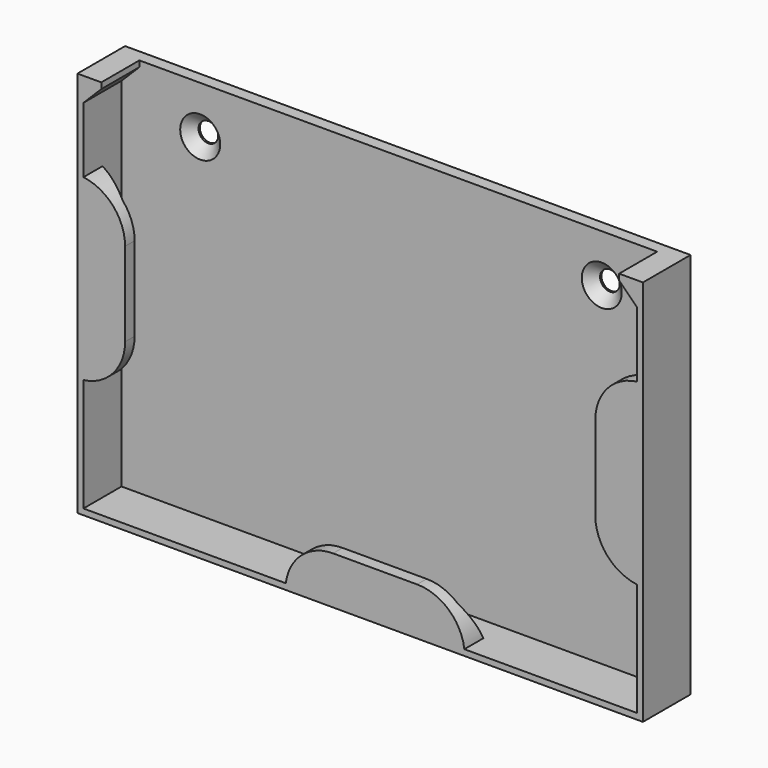
from build123d import *

# Parameters (mm, degrees)
F0_W            = 95
F0_H            = 65
F1_DEPTH        = 10
F2_W            = 93
F2_H            = 63
F3_DEPTH        = 8
F4_W            = 8
F4_H            = 30
F4_W_2          = 30
F4_H_2          = 8
F5_DEPTH        = 2
F6_T1_DEPTH     = 21.843134833
F6_T6_DEPTH     = 41.686269666
F6_T11_DEPTH    = 41.686269666
F7_C1_SIZE2     = 2
F7_C1_SIZE      = 5
F7_C2_SIZE2     = 5
F7_C2_SIZE      = 2
F7_C3_SIZE2     = 2
F7_C3_SIZE      = 5
F8_W            = 87
F8_H            = 8
F9_DEPTH        = 10
F10_SIZE        = 2.99999
F12_D           = 3.3
F12_CSINK_D     = 6.72
F12_CSINK_ANGLE = 90


# Not quite as in the source:
# - a fillet or chamfer that OpenCascade refuses, or shapes differently, is made with other operations: its cross-section is extruded or revolved along the edge and cut away or added
# - a fillet or chamfer is up to 0.001 mm smaller than in the source, because OpenCascade refuses the exact size


with BuildPart() as f1:
    # F0 (on Front) → F1 (new body)
    with BuildSketch(Plane.XZ):
        Rectangle(F0_W, F0_H)
    extrude(amount=F1_DEPTH)

    # F2 (on face) → F3 (cut)
    with BuildSketch(Plane.XZ.offset(10)):
        Rectangle(F2_W, F2_H)
    extrude(amount=-F3_DEPTH, mode=Mode.SUBTRACT)

    # F4 (on face) → F5 (join)
    with BuildSketch(Plane.XZ.offset(10)):
        with Locations((-43.5, 2.5)):
            Rectangle(F4_W, F4_H)
        with Locations((43.5, 2.5)):
            Rectangle(F4_W, F4_H)
        with Locations((2.5, -28.5)):
            Rectangle(F4_W_2, F4_H_2)
    extrude(amount=-F5_DEPTH)

    # F6: fillet of radius 8 on 6 edges, made by hand

    # F6_s2 → F6_t1 (cut)
    with BuildSketch(Plane.XZ.offset(8)):
        with BuildLine():
            ThreePointArc((-39.5, -4.5627460668), (-41.5, -9.8542486889), (-46.5, -12.5))
            Line((-46.5, -12.5), (-39.5, -12.5))
            Line((-39.5, -12.5), (-39.5, -4.5627460668))
        make_face()
        with BuildLine():
            ThreePointArc((-46.5, 17.5), (-41.5, 14.8542486889), (-39.5, 9.5627460668))
            Line((-39.5, 9.5627460668), (-39.5, 17.5))
            Line((-39.5, 17.5), (-46.5, 17.5))
        make_face()
        with BuildLine():
            ThreePointArc((-12.5, -31.5), (-9.8542486889, -26.5), (-4.5627460668, -24.5))
            Line((-4.5627460668, -24.5), (-12.5, -24.5))
            Line((-12.5, -24.5), (-12.5, -31.5))
        make_face()
        with BuildLine():
            ThreePointArc((9.5627460668, -24.5), (14.8542486889, -26.5), (17.5, -31.5))
            Line((17.5, -31.5), (17.5, -24.5))
            Line((17.5, -24.5), (9.5627460668, -24.5))
        make_face()
    extrude(amount=F6_T1_DEPTH, mode=Mode.SUBTRACT)


with BuildPart() as f6_tool4:
    # F6_s5 → F6_t6 (new body)
    with BuildSketch(Plane.XZ.offset(29.843134833)):
        with BuildLine():
            ThreePointArc((39.5, 9.5627460668), (41.5, 14.8542486889), (46.5, 17.5))
            Line((46.5, 17.5), (39.5, 17.5))
            Line((39.5, 17.5), (39.5, 9.5627460668))
        make_face()
    extrude(amount=-F6_T6_DEPTH)

    split(bisect_by=Plane.XZ.offset(2), keep=Keep.TOP)


with BuildPart() as f1_1:
    add(f1.part)

    # F6_t3: cut F6_tool4
    add(f6_tool4.part, mode=Mode.SUBTRACT)


with BuildPart() as f6_tool9:
    # F6_s10 → F6_t11 (new body)
    with BuildSketch(Plane.XZ.offset(29.843134833)):
        with BuildLine():
            ThreePointArc((46.5, -12.5), (41.5, -9.8542486889), (39.5, -4.5627460668))
            Line((39.5, -4.5627460668), (39.5, -12.5))
            Line((39.5, -12.5), (46.5, -12.5))
        make_face()
    extrude(amount=-F6_T11_DEPTH)

    split(bisect_by=Plane.XZ.offset(2), keep=Keep.TOP)


with BuildPart() as f1_2:
    add(f1_1.part)

    # F6_t8: cut F6_tool9
    add(f6_tool9.part, mode=Mode.SUBTRACT)

    # F7: chamfer of 2 x 5 on 3 edges, made by hand

    # F7_c1
    f7_c1_edges = [f1_2.edges().sort_by_distance(p)[0] for p in [
        (2.5, -8, -31.5),
    ]]
    f7_c1_side = f1_2.faces().sort_by_distance((2.5, -8, -31.46))[0]
    chamfer(f7_c1_edges, length=F7_C1_SIZE, length2=F7_C1_SIZE2, reference=f7_c1_side)

    # F7_c2
    f7_c2_edges = [f1_2.edges().sort_by_distance(p)[0] for p in [
        (-46.5, -8, 2.5),
    ]]
    f7_c2_side = f1_2.faces().sort_by_distance((-46.5, -7.96, 2.5))[0]
    chamfer(f7_c2_edges, length=F7_C2_SIZE, length2=F7_C2_SIZE2, reference=f7_c2_side)

    # F7_c3
    f7_c3_edges = [f1_2.edges().sort_by_distance(p)[0] for p in [
        (46.5, -8, 2.5),
    ]]
    f7_c3_side = f1_2.faces().sort_by_distance((46.5, -7.96, 2.5))[0]
    chamfer(f7_c3_edges, length=F7_C3_SIZE, length2=F7_C3_SIZE2, reference=f7_c3_side)

    # F8 (on face) → F9 (cut)
    with BuildSketch(Plane.XY.offset(32.5)):
        with Locations((0, -6)):
            Rectangle(F8_W, F8_H)
    extrude(amount=-F9_DEPTH, mode=Mode.SUBTRACT)

    # F10 (size 3 in the source; OpenCascade refuses exactly that, so slightly less here)
    f10_edges = [f1_2.edges().sort_by_distance(p)[0] for p in [
        (-46.5, -6, 31.5),
        (46.5, -6, 31.5),
    ]]
    chamfer(f10_edges, length=F10_SIZE)

    # F12 (through all)
    with Locations(Plane.XZ.offset(2)):
        with Locations((34.1857404726, 24.5), (-33.2815715389, 24.5)):
            CounterSinkHole(F12_D / 2, F12_CSINK_D / 2, counter_sink_angle=F12_CSINK_ANGLE)


solid = f1_2.part
